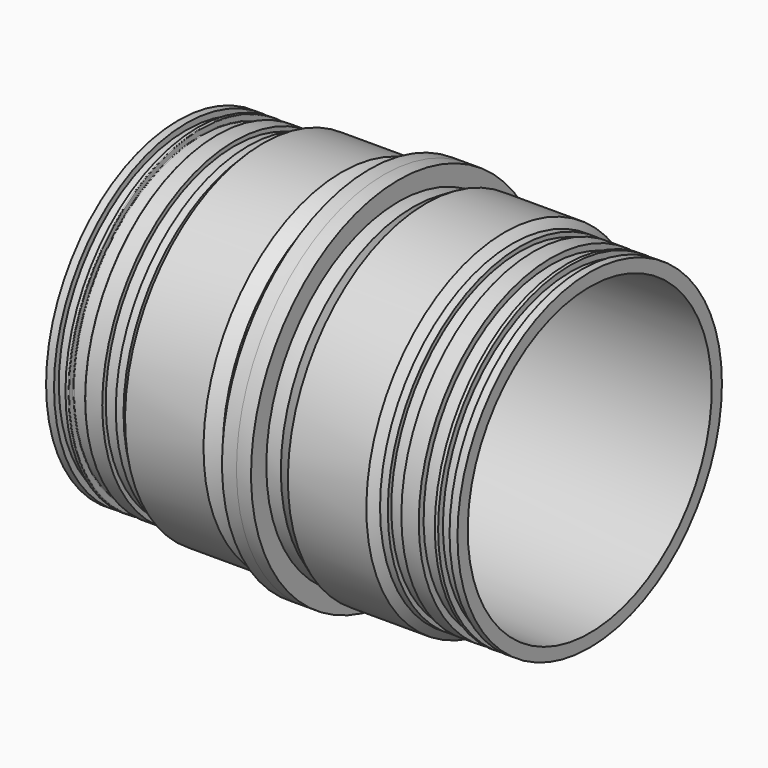
from build123d import *

# Parameters (mm, degrees)
F2_R    = 3.302
F3_SIZE = 12.7


# Not quite as in the source:
# - a pattern or mirror of a feature is missing from the dataset's text; its kind, count and spacing are read off the source's solid


with BuildPart() as f1:
    # F0 (on Front) → F1 (revolve)
    with BuildSketch(Plane.XZ):
        Polygon((41.656, 867.41), (0, 867.41), (0, 800.1), (1079.5, 800.1), (1079.5, 967.74), (1003.3, 967.74), (1003.3, 867.41), (927.1, 867.41), (858.0292778958, 907.288), (446.278, 907.288), (406.4, 867.41), (365.76, 867.41), (365.76, 844.55), (294.64, 844.55), (294.64, 867.41), (203.2, 867.41), (203.2, 835.787), (119.0872639418, 835.787), (119.0872639418, 867.41), (101.6, 867.41), (101.6, 835.787), (41.656, 835.787), align=None)
    revolve(axis=Axis((836.0699839478, 0, 0), (1, 0, 0)))


with BuildPart() as f1_copies_1:
    # F1_copies: instance of F1
    add(f1.part.mirror(Plane(origin=(1079.5, 0, 0), x_dir=(0, 0, 1), z_dir=(1, 0, 0))))


with BuildPart() as f1_1:
    add(f1.part)

    # F2
    f2_edges = [f1_1.edges().sort_by_distance(p)[0] for p in [
        (203.2, 0, -867.41),
        (203.2, 0, -835.787),
        (119.087264, 0, -867.41),
        (119.087264, 0, -835.787),
    ]]
    fillet(f2_edges, radius=F2_R)

    # F3
    f3_edges = [f1_1.edges().sort_by_distance(p)[0] for p in [
        (365.76, 0, -844.55),
    ]]
    chamfer(f3_edges, length=F3_SIZE)


solid = Compound([f1_copies_1.part, f1_1.part])
